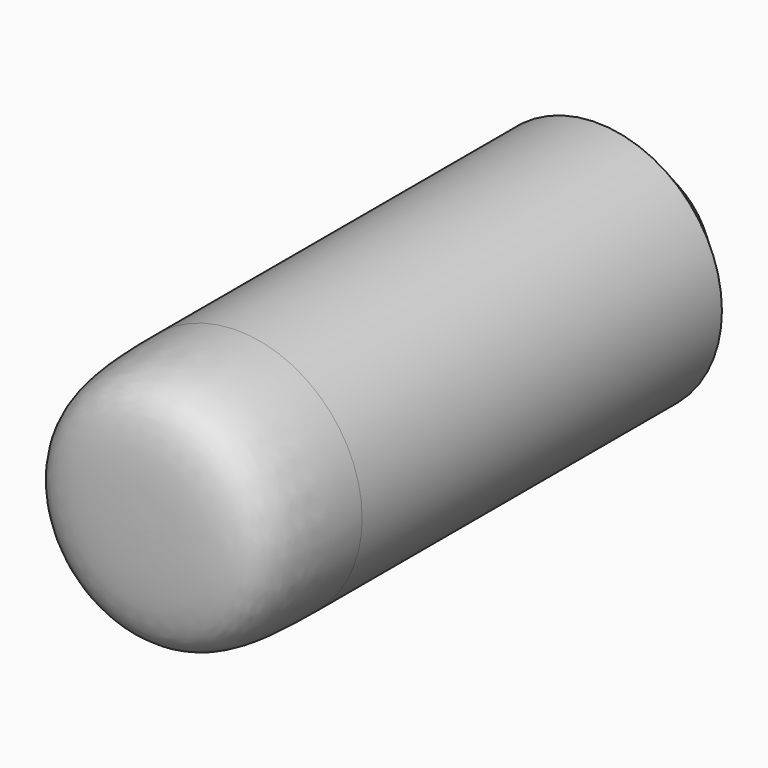
from build123d import *

# Parameters (mm, degrees)
F0_R     = 12.7
F1_DEPTH = 63.5
F2_SIZE  = 5.08


# Not quite as in the source:
# - a fillet or chamfer that OpenCascade refuses, or shapes differently, is made with other operations: its cross-section is extruded or revolved along the edge and cut away or added


with BuildPart() as f1:
    # F0 (on Front) → F1 (new body)
    with BuildSketch(Plane.XZ):
        Circle(F0_R)
    extrude(amount=F1_DEPTH)

    # F2
    f2_edges = [f1.edges().sort_by_distance(p)[0] for p in [
        (-12.7, 0, 0),
    ]]
    chamfer(f2_edges, length=F2_SIZE)

    # F3: fillet of radius 12.7 on 1 edges, made by hand

    # F3_s1 → F3_t2 (revolve, cut)
    with BuildSketch(Plane.XY):
        with BuildLine():
            add(Edge.make_bspline(
                [(12.7, -50.8), (12.7, -63.5), (0, -63.5)],
                knots=[0, 0, 0, 1, 1, 1], degree=2, weights=[1, 2.3333333333, 1]))
            Line((0, -63.5), (12.7, -63.5))
            Line((12.7, -63.5), (12.7, -50.8))
        make_face()
    revolve(axis=Axis((0, -63.5, 0), (0, -1, 0)), mode=Mode.SUBTRACT)


solid = f1.part
